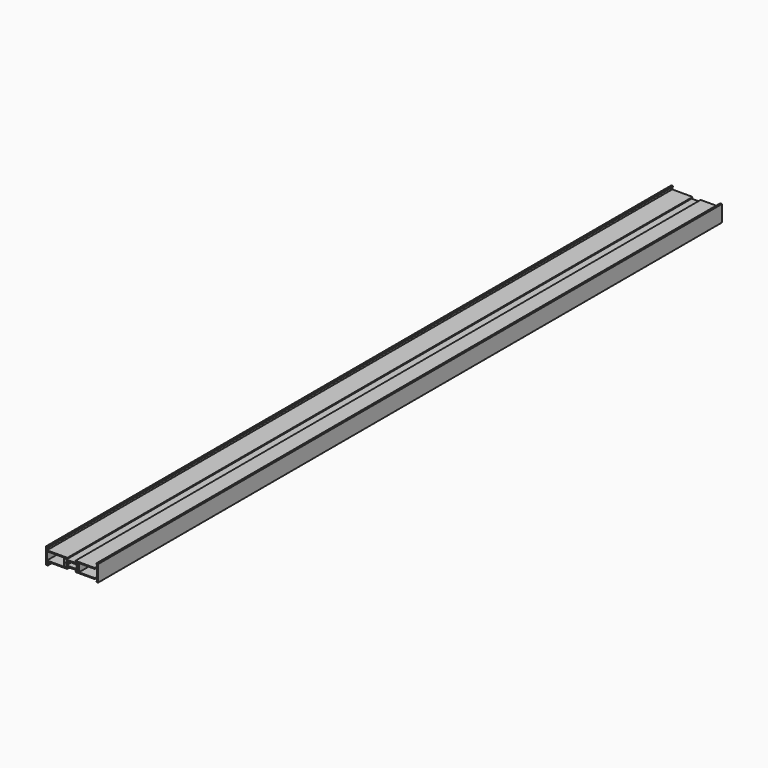
from build123d import *

# Parameters (mm, degrees)
F1_DEPTH = 1300
F0_W     = 27.9218892101
F0_H     = 13.4031483904
F3_DEPTH = 3


with BuildPart() as f1:
    # F0 (on Front) → F1 (new body)
    with BuildSketch(Plane.XZ):
        Polygon((33.1643968821, 8.8389720768), (35.3255756199, 10.1125258952), (51.900004968, 10.1125258952), (54.0555718382, 8.8389720768), (54.0555718382, 12.7773806453), (53.6706149578, 12.7773806453), (51.900004968, 11.8849426508), (35.3255756199, 11.8849426508), (33.6281075799, 12.8878421359), (33.1643968821, 12.8878421359), align=None)
    extrude(amount=F1_DEPTH)


with BuildPart() as f1b:
    # F0 (on Front) → F1, piece 2 (new body)
    with BuildSketch(Plane.XZ):
        with BuildLine():
            ThreePointArc((1.7400689467, 28.9004424067), (1.610154442, 28.8458538917), (1.5564486384, 28.7155720005))
            Line((1.5564486384, 28.7155720005), (1.5564486384, 1.7487789137))
            ThreePointArc((1.5564486384, 1.7487789137), (1.6189816628, 1.5978108381), (1.7699497384, 1.5352778137))
            Line((1.7699497384, 1.5352778137), (4.3837734866, 1.5352778137))
            ThreePointArc((4.3837734866, 1.5352778137), (4.5347415622, 1.5978108381), (4.5972745866, 1.7487789137))
            Line((4.5972745866, 1.7487789137), (4.5972745866, 2.8025670345))
            ThreePointArc((4.5972745866, 2.8025670345), (4.5347415622, 2.9535351101), (4.3837734866, 3.0160681345))
            Line((4.3837734866, 3.0160681345), (3.2995220372, 3.0160681345))
            ThreePointArc((3.2995220372, 3.0160681345), (3.1485539616, 3.0786011589), (3.0860209372, 3.2295692345))
            Line((3.0860209372, 3.2295692345), (3.0860209372, 6.73822727))
            ThreePointArc((3.0860209372, 6.73822727), (3.1485539616, 6.8891953456), (3.2995220372, 6.95172837))
            Line((3.2995220372, 6.95172837), (36.7220732833, 6.95172837))
            ThreePointArc((36.7220732833, 6.95172837), (36.909094242, 7.0622446134), (36.9024969591, 7.2793785695))
            Line((36.9024969591, 7.2793785695), (35.4109538688, 9.6369064715))
            ThreePointArc((35.4109538688, 9.6369064715), (35.2864431086, 9.7288070398), (35.1325563369, 9.7124514501))
            Line((35.1325563369, 9.7124514501), (33.3064083824, 8.7692762138))
            ThreePointArc((33.3064083824, 8.7692762138), (33.0973823007, 8.7766241296), (32.9949334264, 8.9589702918))
            Line((32.9949334264, 8.9589702918), (32.9949334264, 13.052558215))
            ThreePointArc((32.9949334264, 13.052558215), (33.1065923516, 13.2402038682), (33.3247761404, 13.2315759475))
            Line((33.3247761404, 13.2315759475), (35.1508547592, 12.0448279597))
            ThreePointArc((35.1508547592, 12.0448279597), (35.266845262, 12.0402411989), (35.326205194, 12.1399970688))
            Line((35.326205194, 12.1399970688), (35.326205194, 14.1000744849))
            ThreePointArc((35.326205194, 14.1000744849), (35.3120005783, 14.1550536436), (35.2729421347, 14.1962715644))
            Line((35.2729421347, 14.1962715644), (34.0620617039, 14.954517704))
            ThreePointArc((34.0620617039, 14.954517704), (33.9622249211, 15.1231859929), (34.0420253617, 15.3022062838))
            Line((34.0420253617, 15.3022062838), (35.2835938216, 16.2951429765))
            ThreePointArc((35.2835938216, 16.2951429765), (35.3149991617, 16.334608133), (35.326205194, 16.3837835213))
            Line((35.326205194, 16.3837835213), (35.326205194, 18.2900932618))
            ThreePointArc((35.326205194, 18.2900932618), (35.2692768061, 18.3884905579), (35.1555984257, 18.3881822121))
            Line((35.1555984257, 18.3881822121), (33.5908916097, 17.4772373113))
            ThreePointArc((33.5908916097, 17.4772373113), (33.5633603883, 17.4657459183), (33.5337859409, 17.4618251622))
            Line((33.5337859409, 17.4618251622), (33.1084345259, 17.4618251622))
            ThreePointArc((33.1084345259, 17.4618251622), (33.0281771288, 17.4950688645), (32.9949334264, 17.5753262617))
            Line((32.9949334264, 17.5753262617), (32.9949334264, 21.7697896372))
            ThreePointArc((32.9949334264, 21.7697896372), (33.0521783263, 21.8683682333), (33.1661694697, 21.8675095219))
            Line((33.1661694697, 21.8675095219), (35.2315651953, 20.6472306944))
            ThreePointArc((35.2315651953, 20.6472306944), (35.3158103776, 20.6345888698), (35.3851216132, 20.6841168326))
            Line((35.3851216132, 20.6841168326), (36.9991130564, 23.2263741871))
            ThreePointArc((36.9991130564, 23.2263741871), (37.0027581513, 23.341878778), (36.9032915823, 23.400709033))
            Line((36.9032915823, 23.400709033), (3.1995220367, 23.400709033))
            ThreePointArc((3.1995220367, 23.400709033), (3.1192646396, 23.4339527354), (3.0860209372, 23.5142101325))
            Line((3.0860209372, 23.5142101325), (3.0860209372, 27.3130099498))
            ThreePointArc((3.0860209372, 27.3130099498), (3.1192646396, 27.3932673469), (3.1995220367, 27.4265110493))
            Line((3.1995220367, 27.4265110493), (4.4884980865, 27.4265110493))
            ThreePointArc((4.4884980865, 27.4265110493), (4.5687554836, 27.4597547517), (4.601999186, 27.5400121488))
            Line((4.601999186, 27.5400121488), (4.601999186, 28.8055868989))
            ThreePointArc((4.601999186, 28.8055868989), (4.5684827516, 28.8861161044), (4.4877279946, 28.9190853859))
            Line((4.4877279946, 28.9190853859), (1.7400689467, 28.9004424067))
        make_face()
        with Locations((17.0469655422, 15.1840499602)):
            Rectangle(F0_W, F0_H, mode=Mode.SUBTRACT)
    extrude(amount=F1_DEPTH)


with BuildPart() as f1c:
    # F0 (on Front) → F1, piece 3 (new body)
    with BuildSketch(Plane.XZ):
        with BuildLine():
            Line((54.1477753989, 17.4618251622), (53.7224239839, 17.4618251622))
            ThreePointArc((53.7224239839, 17.4618251622), (53.6928495365, 17.4657459183), (53.6653183151, 17.4772373113))
            Line((53.6653183151, 17.4772373113), (52.1006114991, 18.3881822121))
            ThreePointArc((52.1006114991, 18.3881822121), (51.9869331187, 18.3884905579), (51.9300047308, 18.2900932618))
            Line((51.9300047308, 18.2900932618), (51.9300047308, 16.3837835213))
            ThreePointArc((51.9300047308, 16.3837835213), (51.9412107631, 16.334608133), (51.9726161032, 16.2951429765))
            Line((51.9726161032, 16.2951429765), (53.2141845631, 15.3022062838))
            ThreePointArc((53.2141845631, 15.3022062838), (53.2939850037, 15.1231859929), (53.1941482209, 14.954517704))
            Line((53.1941482209, 14.954517704), (51.9832677901, 14.1962715644))
            ThreePointArc((51.9832677901, 14.1962715644), (51.9442093465, 14.1550536436), (51.9300047308, 14.1000744849))
            Line((51.9300047308, 14.1000744849), (51.9300047308, 12.1399970688))
            ThreePointArc((51.9300047308, 12.1399970688), (51.9893646628, 12.0402411989), (52.1053551656, 12.0448279597))
            Line((52.1053551656, 12.0448279597), (53.9314337844, 13.2315759475))
            ThreePointArc((53.9314337844, 13.2315759475), (54.1496175732, 13.2402038682), (54.2612764984, 13.052558215))
            Line((54.2612764984, 13.052558215), (54.2612764984, 8.9589702918))
            ThreePointArc((54.2612764984, 8.9589702918), (54.1588276241, 8.7766241296), (53.9498015424, 8.7692762138))
            Line((53.9498015424, 8.7692762138), (52.1236535879, 9.7124514501))
            ThreePointArc((52.1236535879, 9.7124514501), (51.9697668162, 9.7288070398), (51.845256056, 9.6369064715))
            Line((51.845256056, 9.6369064715), (50.3537129657, 7.2793785695))
            ThreePointArc((50.3537129657, 7.2793785695), (50.3471156828, 7.0622446134), (50.5341366415, 6.95172837))
            Line((50.5341366415, 6.95172837), (83.9566878876, 6.95172837))
            ThreePointArc((83.9566878876, 6.95172837), (84.1076559632, 6.8891953456), (84.1701889876, 6.73822727))
            Line((84.1701889876, 6.73822727), (84.1701889876, 3.2295692345))
            ThreePointArc((84.1701889876, 3.2295692345), (84.1076559632, 3.0786011589), (83.9566878876, 3.0160681345))
            Line((83.9566878876, 3.0160681345), (82.8724364383, 3.0160681345))
            ThreePointArc((82.8724364383, 3.0160681345), (82.7214683627, 2.9535351101), (82.6589353383, 2.8025670345))
            Line((82.6589353383, 2.8025670345), (82.6589353383, 1.7487789137))
            ThreePointArc((82.6589353383, 1.7487789137), (82.7214683627, 1.5978108381), (82.8724364383, 1.5352778137))
            Line((82.8724364383, 1.5352778137), (85.4862601864, 1.5352778137))
            ThreePointArc((85.4862601864, 1.5352778137), (85.637228262, 1.5978108381), (85.6997612864, 1.7487789137))
            Line((85.6997612864, 1.7487789137), (85.6997612864, 28.7155720005))
            ThreePointArc((85.6997612864, 28.7155720005), (85.6460554828, 28.8458538917), (85.5161409781, 28.9004424067))
            Line((85.5161409781, 28.9004424067), (82.7684819302, 28.9190853859))
            ThreePointArc((82.7684819302, 28.9190853859), (82.6877271732, 28.8861161044), (82.6542107388, 28.8055868989))
            Line((82.6542107388, 28.8055868989), (82.6542107388, 27.5400121488))
            ThreePointArc((82.6542107388, 27.5400121488), (82.6874544412, 27.4597547516), (82.7677118384, 27.4265110493))
            Line((82.7677118384, 27.4265110493), (84.0566878881, 27.4265110493))
            ThreePointArc((84.0566878881, 27.4265110493), (84.1369452853, 27.3932673469), (84.1701889876, 27.3130099498))
            Line((84.1701889876, 27.3130099498), (84.1701889876, 23.5142101325))
            ThreePointArc((84.1701889876, 23.5142101325), (84.1369452853, 23.4339527354), (84.0566878881, 23.400709033))
            Line((84.0566878881, 23.400709033), (50.3529183425, 23.400709033))
            ThreePointArc((50.3529183425, 23.400709033), (50.2534517735, 23.341878778), (50.2570968685, 23.2263741871))
            Line((50.2570968685, 23.2263741871), (51.8710883117, 20.6841168326))
            ThreePointArc((51.8710883117, 20.6841168326), (51.9403995472, 20.6345888698), (52.0246447296, 20.6472306944))
            Line((52.0246447296, 20.6472306944), (54.0900404551, 21.8675095219))
            ThreePointArc((54.0900404551, 21.8675095219), (54.2040315985, 21.8683682333), (54.2612764984, 21.7697896372))
            Line((54.2612764984, 21.7697896372), (54.2612764984, 17.5753262617))
            ThreePointArc((54.2612764984, 17.5753262617), (54.2280327961, 17.4950688645), (54.1477753989, 17.4618251622))
        make_face()
        with Locations((70.2092443826, 15.1840499602)):
            Rectangle(F0_W, F0_H, mode=Mode.SUBTRACT)
    extrude(amount=F1_DEPTH)

    # F2 (on face) → F3 (cut)
    with BuildSketch(Plane.XZ.offset(1300)):
        with BuildLine():
            Line((84.0566878881, 23.400709033), (82.6542107388, 23.400709033))
            Line((82.6542107388, 23.400709033), (82.6542107388, 21.8856241554))
            Line((82.6542107388, 21.8856241554), (84.1701889876, 21.8856241554))
            Line((84.1701889876, 21.8856241554), (84.1701889876, 8.482475765))
            Line((84.1701889876, 8.482475765), (82.6542107388, 8.482475765))
            Line((82.6542107388, 8.482475765), (82.6542107388, 6.95172837))
            Line((82.6542107388, 6.95172837), (83.9566878876, 6.95172837))
            ThreePointArc((83.9566878876, 6.95172837), (84.1076559632, 6.8891953456), (84.1701889876, 6.73822727))
            Line((84.1701889876, 6.73822727), (84.1701889876, 3.2295692345))
            ThreePointArc((84.1701889876, 3.2295692345), (84.1076559632, 3.0786011589), (83.9566878876, 3.0160681345))
            Line((83.9566878876, 3.0160681345), (82.8724364383, 3.0160681345))
            ThreePointArc((82.8724364383, 3.0160681345), (82.7214683627, 2.9535351101), (82.6589353383, 2.8025670345))
            Line((82.6589353383, 2.8025670345), (82.6589353383, 1.7487789137))
            ThreePointArc((82.6589353383, 1.7487789137), (82.7214683627, 1.5978108381), (82.8724364383, 1.5352778137))
            Line((82.8724364383, 1.5352778137), (85.4862601864, 1.5352778137))
            ThreePointArc((85.4862601864, 1.5352778137), (85.637228262, 1.5978108381), (85.6997612864, 1.7487789137))
            Line((85.6997612864, 1.7487789137), (85.6997612864, 28.7155720005))
            ThreePointArc((85.6997612864, 28.7155720005), (85.6460554828, 28.8458538917), (85.5161409781, 28.9004424067))
            Line((85.5161409781, 28.9004424067), (82.7684819302, 28.9190853859))
            ThreePointArc((82.7684819302, 28.9190853859), (82.6877271732, 28.8861161044), (82.6542107388, 28.8055868989))
            Line((82.6542107388, 28.8055868989), (82.6542107388, 27.5400121488))
            ThreePointArc((82.6542107388, 27.5400121488), (82.6874544412, 27.4597547516), (82.7677118384, 27.4265110493))
            Line((82.7677118384, 27.4265110493), (84.0566878881, 27.4265110493))
            ThreePointArc((84.0566878881, 27.4265110493), (84.1369452853, 27.3932673469), (84.1701889876, 27.3130099498))
            Line((84.1701889876, 27.3130099498), (84.1701889876, 23.5142101325))
            ThreePointArc((84.1701889876, 23.5142101325), (84.1369452853, 23.4339527354), (84.0566878881, 23.400709033))
        make_face()
    extrude(amount=-F3_DEPTH, mode=Mode.SUBTRACT)


with BuildPart() as f1d:
    # F0 (on Front) → F1, piece 4 (new body)
    with BuildSketch(Plane.XZ):
        Polygon((35.3555753827, 20.3506425023), (33.1943966448, 21.6241963208), (33.1943966448, 17.5753262617), (33.6581073427, 17.5753262617), (35.3555753827, 18.5782257468), (51.9300047308, 18.5782257468), (53.7006147206, 17.6857877523), (54.0855716009, 17.6857877523), (54.0855716009, 21.6241963208), (51.9300047308, 20.3506425023), align=None)
    extrude(amount=F1_DEPTH)


solid = Compound([f1.part, f1b.part, f1c.part, f1d.part])
